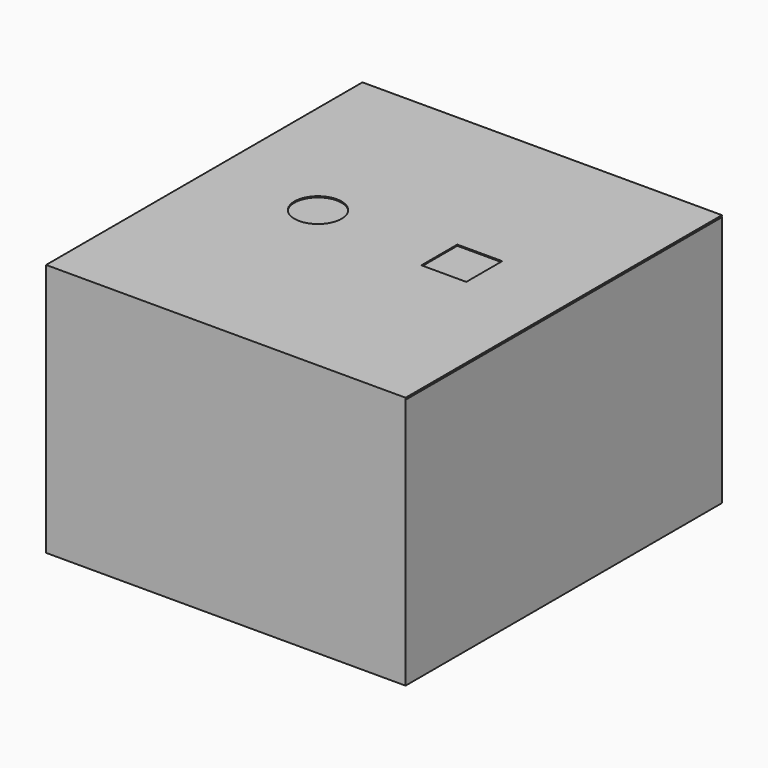
from build123d import *

# Parameters (mm, degrees)
F1_DEPTH = 63.5
F2_W     = 15.875
F2_H     = 15.875
F3_DEPTH = 0.4064


# Not quite as in the source:
# - the dataset's text gives a spline's control points without its knots; the knots are read off the source's solid


with BuildPart() as f1:
    # F0 (on Right) → F1 (new body, symmetric)
    with BuildSketch(Plane.YZ):
        Polygon((-139.7, 0), (0, 0), (0, 88.9), (-139.2936, 88.9), (-139.2936, 89.154), (0, 89.154), (0, 89.5604), (-139.7, 89.5604), align=None)
    extrude(amount=F1_DEPTH, both=True)

    # F2 (on face) → F3 (cut, through all)
    with BuildSketch(Plane.XY.offset(89.5604)):
        with Locations((25.4164397061, -67.2669539907)):
            Rectangle(F2_W, F2_H)
        with BuildLine():
            add(Edge.make_bspline(
                [(-19.4903538939, -61.3735951907), (-21.0330482939, -59.8307229907), (-23.2013954939, -58.9325789907), (-25.3835602939, -58.9325789907)],
                knots=[7, 7, 7, 7, 8, 8, 8, 8], degree=3))
            add(Edge.make_bspline(
                [(-25.3835602939, -58.9325789907), (-27.5652932939, -58.9325789907), (-29.7339960939, -59.8307229907), (-31.2766904939, -61.3735951907)],
                knots=[0, 0, 0, 0, 1, 1, 1, 1], degree=3))
            add(Edge.make_bspline(
                [(-31.2766904939, -61.3735951907), (-32.8194356939, -62.9164927907), (-33.7179352939, -65.0849923907), (-33.7179352939, -67.2669539907), (-33.7179352939, -69.4487377907), (-32.8194356939, -71.6174151907), (-31.2766904939, -73.1601603907)],
                knots=[1, 1, 1, 1, 2, 2, 2, 3, 3, 3, 3], degree=3))
            add(Edge.make_bspline(
                [(-31.2766904939, -73.1601603907), (-29.7339960939, -74.7032103907), (-27.5652932939, -75.6013289907), (-25.3835602939, -75.6013289907), (-23.2013954939, -75.6013289907), (-21.0330482939, -74.7032103907), (-19.4903538939, -73.1601603907)],
                knots=[3, 3, 3, 3, 4, 4, 4, 5, 5, 5, 5], degree=3))
            add(Edge.make_bspline(
                [(-19.4903538939, -73.1601603907), (-17.9473038939, -71.6174151907), (-17.0491852939, -69.4487377907), (-17.0491852939, -67.2669539907), (-17.0491852939, -65.0849923907), (-17.9473038939, -62.9164927907), (-19.4903538939, -61.3735951907)],
                knots=[5, 5, 5, 5, 6, 6, 6, 7, 7, 7, 7], degree=3))
        make_face()
    extrude(amount=-F3_DEPTH, mode=Mode.SUBTRACT)


solid = f1.part
